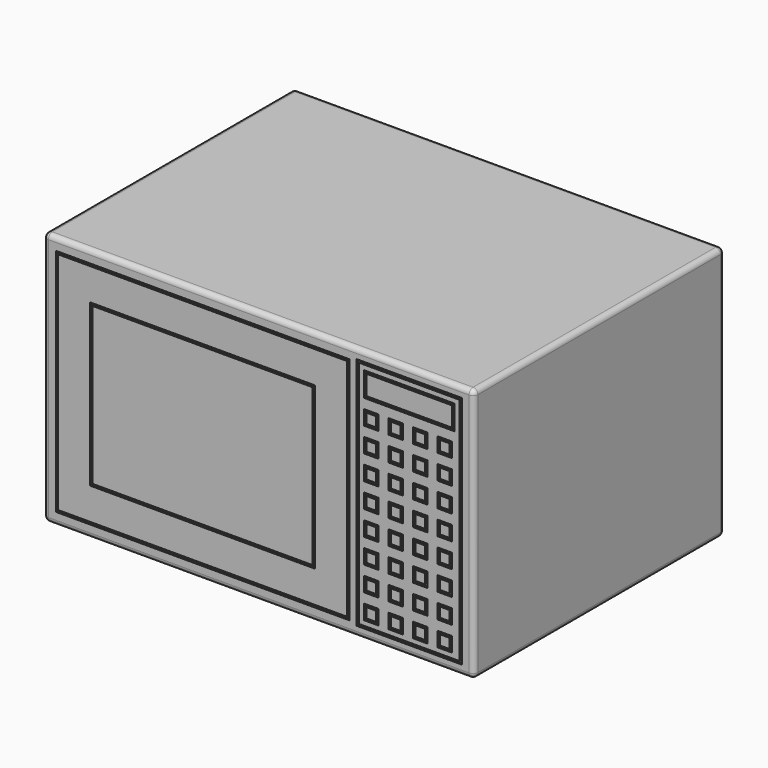
from build123d import *

# Parameters (mm, degrees)
F0_W                   = 558.8
F0_H                   = 330.2
F1_DEPTH               = 406.4
F2_R                   = 6.35
F3_W                   = 342.9
F3_H                   = 215.9
F4_DEPTH               = 50.8
DRAFT_F4_DRAFTED_ANGLE = 30
F5_R                   = 38.1
F6_W                   = 381
F6_H                   = 298.45
F6_W_2                 = 374.65
F6_H_2                 = 292.1
F6_W_3                 = 292.1
F6_H_3                 = 209.55
F6_W_4                 = 285.75
F6_H_4                 = 203.2
F6_W_5                 = 136.525
F6_H_5                 = 304.8
F6_W_6                 = 130.175
F6_W_7                 = 117.475
F6_H_6                 = 31.75
F6_W_8                 = 111.125
F6_H_7                 = 25.4
F6_W_9                 = 19.05
F6_H_8                 = 19.05
F6_W_10                = 12.7
F6_H_9                 = 12.7
F7_DEPTH               = 3.175


# Not quite as in the source:
# - an extrude with a draft is written as a straight extrude whose walls are then drafted


with BuildPart() as f1:
    # F0 (on Front) → F1 (new body)
    with BuildSketch(Plane.XZ):
        with Locations((-279.4, 165.1)):
            Rectangle(F0_W, F0_H)
    extrude(amount=-F1_DEPTH)

    # F2
    f2_edges = [f1.edges().sort_by_distance(p)[0] for p in [
        (0, 203.2, 330.2),
        (-558.8, 203.2, 330.2),
        (-279.4, 0, 330.2),
        (-279.4, 406.4, 330.2),
        (0, 203.2, 0),
        (0, 0, 165.1),
        (0, 406.4, 165.1),
        (-279.4, 406.4, 0),
        (-558.8, 406.4, 165.1),
        (-279.4, 0, 0),
        (-558.8, 0, 165.1),
        (-558.8, 203.2, 0),
    ]]
    fillet(f2_edges, radius=F2_R)


with BuildPart() as f4_drafted:
    # F3 (on face) → F4 (new body)
    with BuildSketch(Plane(origin=(0, 406.4, 0), x_dir=(-1, 0, 0), z_dir=(0, 1, 0))):
        with Locations((336.55, 171.45)):
            Rectangle(F3_W, F3_H)
    extrude(amount=F4_DEPTH)

    # draft_F4_drafted
    draft_f4_drafted_walls = [f4_drafted.faces().sort_by_distance(p)[0] for p in [
        (-336.55, 440.2666666667, 63.5),
        (-508, 440.2666666667, 171.45),
        (-336.55, 440.2666666667, 279.4),
        (-165.1, 440.2666666667, 171.45),
    ]]
    draft(draft_f4_drafted_walls, neutral_plane=Plane(origin=(0, 406.4, 0), x_dir=(-1, 0, 0), z_dir=(0, 1, 0)), angle=DRAFT_F4_DRAFTED_ANGLE)


with BuildPart() as f1_1:
    add(f1.part)

    # join_F4_drafted: union F4_drafted
    add(f4_drafted.part)

    # F5
    f5_edges = [f1_1.edges().sort_by_distance(p)[0] for p in [
        (-336.55, 457.2, 92.829394),
        (-478.670606, 457.2, 171.45),
        (-336.55, 457.2, 250.070606),
        (-194.429394, 457.2, 171.45),
        (-336.55, 406.4, 279.4),
        (-508, 406.4, 171.45),
        (-165.1, 406.4, 171.45),
        (-336.55, 406.4, 63.5),
    ]]
    fillet(f5_edges, radius=F5_R)

    # F6 (on face) → F7 (cut)
    with BuildSketch(Plane.XZ):
        with Locations((-352.425, 165.1)):
            Rectangle(F6_W, F6_H)
        with Locations((-352.425, 165.1)):
            Rectangle(F6_W_2, F6_H_2, mode=Mode.SUBTRACT)
        with Locations((-352.425, 165.1)):
            Rectangle(F6_W_3, F6_H_3)
        with Locations((-352.425, 165.1)):
            Rectangle(F6_W_4, F6_H_4, mode=Mode.SUBTRACT)
        with Locations((-84.1375, 165.1)):
            Rectangle(F6_W_5, F6_H_5)
        with Locations((-84.1375, 165.1)):
            Rectangle(F6_W_6, F6_H, mode=Mode.SUBTRACT)
        with Locations((-84.1375, 292.1)):
            Rectangle(F6_W_7, F6_H_6)
        with Locations((-84.1375, 292.1)):
            Rectangle(F6_W_8, F6_H_7, mode=Mode.SUBTRACT)
        with Locations((-133.35, 254)):
            Rectangle(F6_W_9, F6_H_8)
        with Locations((-133.35, 254)):
            Rectangle(F6_W_10, F6_H_9, mode=Mode.SUBTRACT)
        with Locations((-101.6, 254)):
            Rectangle(F6_W_9, F6_H_8)
        with Locations((-101.6, 254)):
            Rectangle(F6_W_10, F6_H_9, mode=Mode.SUBTRACT)
        with Locations((-69.85, 254)):
            Rectangle(F6_W_9, F6_H_8)
        with Locations((-69.85, 254)):
            Rectangle(F6_W_10, F6_H_9, mode=Mode.SUBTRACT)
        with Locations((-38.1, 254)):
            Rectangle(F6_W_9, F6_H_8)
        with Locations((-38.1, 254)):
            Rectangle(F6_W_10, F6_H_9, mode=Mode.SUBTRACT)
        with Locations((-38.1, 222.25)):
            Rectangle(F6_W_9, F6_H_8)
        with Locations((-38.1, 222.25)):
            Rectangle(F6_W_10, F6_H_9, mode=Mode.SUBTRACT)
        with Locations((-69.85, 222.25)):
            Rectangle(F6_W_9, F6_H_8)
        with Locations((-69.85, 222.25)):
            Rectangle(F6_W_10, F6_H_9, mode=Mode.SUBTRACT)
        with Locations((-101.6, 222.25)):
            Rectangle(F6_W_9, F6_H_8)
        with Locations((-101.6, 222.25)):
            Rectangle(F6_W_10, F6_H_9, mode=Mode.SUBTRACT)
        with Locations((-133.35, 222.25)):
            Rectangle(F6_W_9, F6_H_8)
        with Locations((-133.35, 222.25)):
            Rectangle(F6_W_10, F6_H_9, mode=Mode.SUBTRACT)
        with Locations((-133.35, 190.5)):
            Rectangle(F6_W_9, F6_H_8)
        with Locations((-133.35, 190.5)):
            Rectangle(F6_W_10, F6_H_9, mode=Mode.SUBTRACT)
        with Locations((-101.6, 190.5)):
            Rectangle(F6_W_9, F6_H_8)
        with Locations((-101.6, 190.5)):
            Rectangle(F6_W_10, F6_H_9, mode=Mode.SUBTRACT)
        with Locations((-69.85, 190.5)):
            Rectangle(F6_W_9, F6_H_8)
        with Locations((-69.85, 190.5)):
            Rectangle(F6_W_10, F6_H_9, mode=Mode.SUBTRACT)
        with Locations((-38.1, 190.5)):
            Rectangle(F6_W_9, F6_H_8)
        with Locations((-38.1, 190.5)):
            Rectangle(F6_W_10, F6_H_9, mode=Mode.SUBTRACT)
        with Locations((-133.35, 158.75)):
            Rectangle(F6_W_9, F6_H_8)
        with Locations((-133.35, 158.75)):
            Rectangle(F6_W_10, F6_H_9, mode=Mode.SUBTRACT)
        with Locations((-101.6, 158.75)):
            Rectangle(F6_W_9, F6_H_8)
        with Locations((-101.6, 158.75)):
            Rectangle(F6_W_10, F6_H_9, mode=Mode.SUBTRACT)
        with Locations((-69.85, 158.75)):
            Rectangle(F6_W_9, F6_H_8)
        with Locations((-69.85, 158.75)):
            Rectangle(F6_W_10, F6_H_9, mode=Mode.SUBTRACT)
        with Locations((-38.1, 158.75)):
            Rectangle(F6_W_9, F6_H_8)
        with Locations((-38.1, 158.75)):
            Rectangle(F6_W_10, F6_H_9, mode=Mode.SUBTRACT)
        with Locations((-38.1, 127)):
            Rectangle(F6_W_9, F6_H_8)
        with Locations((-38.1, 127)):
            Rectangle(F6_W_10, F6_H_9, mode=Mode.SUBTRACT)
        with Locations((-69.85, 127)):
            Rectangle(F6_W_9, F6_H_8)
        with Locations((-69.85, 127)):
            Rectangle(F6_W_10, F6_H_9, mode=Mode.SUBTRACT)
        with Locations((-101.6, 127)):
            Rectangle(F6_W_9, F6_H_8)
        with Locations((-101.6, 127)):
            Rectangle(F6_W_10, F6_H_9, mode=Mode.SUBTRACT)
        with Locations((-133.35, 127)):
            Rectangle(F6_W_9, F6_H_8)
        with Locations((-133.35, 127)):
            Rectangle(F6_W_10, F6_H_9, mode=Mode.SUBTRACT)
        with Locations((-133.35, 95.25)):
            Rectangle(F6_W_9, F6_H_8)
        with Locations((-133.35, 95.25)):
            Rectangle(F6_W_10, F6_H_9, mode=Mode.SUBTRACT)
        with Locations((-101.6, 95.25)):
            Rectangle(F6_W_9, F6_H_8)
        with Locations((-101.6, 95.25)):
            Rectangle(F6_W_10, F6_H_9, mode=Mode.SUBTRACT)
        with Locations((-69.85, 95.25)):
            Rectangle(F6_W_9, F6_H_8)
        with Locations((-69.85, 95.25)):
            Rectangle(F6_W_10, F6_H_9, mode=Mode.SUBTRACT)
        with Locations((-38.1, 95.25)):
            Rectangle(F6_W_9, F6_H_8)
        with Locations((-38.1, 95.25)):
            Rectangle(F6_W_10, F6_H_9, mode=Mode.SUBTRACT)
        with Locations((-38.1, 63.5)):
            Rectangle(F6_W_9, F6_H_8)
        with Locations((-38.1, 63.5)):
            Rectangle(F6_W_10, F6_H_9, mode=Mode.SUBTRACT)
        with Locations((-69.85, 63.5)):
            Rectangle(F6_W_9, F6_H_8)
        with Locations((-69.85, 63.5)):
            Rectangle(F6_W_10, F6_H_9, mode=Mode.SUBTRACT)
        with Locations((-101.6, 63.5)):
            Rectangle(F6_W_9, F6_H_8)
        with Locations((-101.6, 63.5)):
            Rectangle(F6_W_10, F6_H_9, mode=Mode.SUBTRACT)
        with Locations((-133.35, 63.5)):
            Rectangle(F6_W_9, F6_H_8)
        with Locations((-133.35, 63.5)):
            Rectangle(F6_W_10, F6_H_9, mode=Mode.SUBTRACT)
        with Locations((-133.35, 31.75)):
            Rectangle(F6_W_9, F6_H_8)
        with Locations((-133.35, 31.75)):
            Rectangle(F6_W_10, F6_H_9, mode=Mode.SUBTRACT)
        with Locations((-101.6, 31.75)):
            Rectangle(F6_W_9, F6_H_8)
        with Locations((-101.6, 31.75)):
            Rectangle(F6_W_10, F6_H_9, mode=Mode.SUBTRACT)
        with Locations((-69.85, 31.75)):
            Rectangle(F6_W_9, F6_H_8)
        with Locations((-69.85, 31.75)):
            Rectangle(F6_W_10, F6_H_9, mode=Mode.SUBTRACT)
        with Locations((-38.1, 31.75)):
            Rectangle(F6_W_9, F6_H_8)
        with Locations((-38.1, 31.75)):
            Rectangle(F6_W_10, F6_H_9, mode=Mode.SUBTRACT)
    extrude(amount=-F7_DEPTH, mode=Mode.SUBTRACT)


solid = f1_1.part
